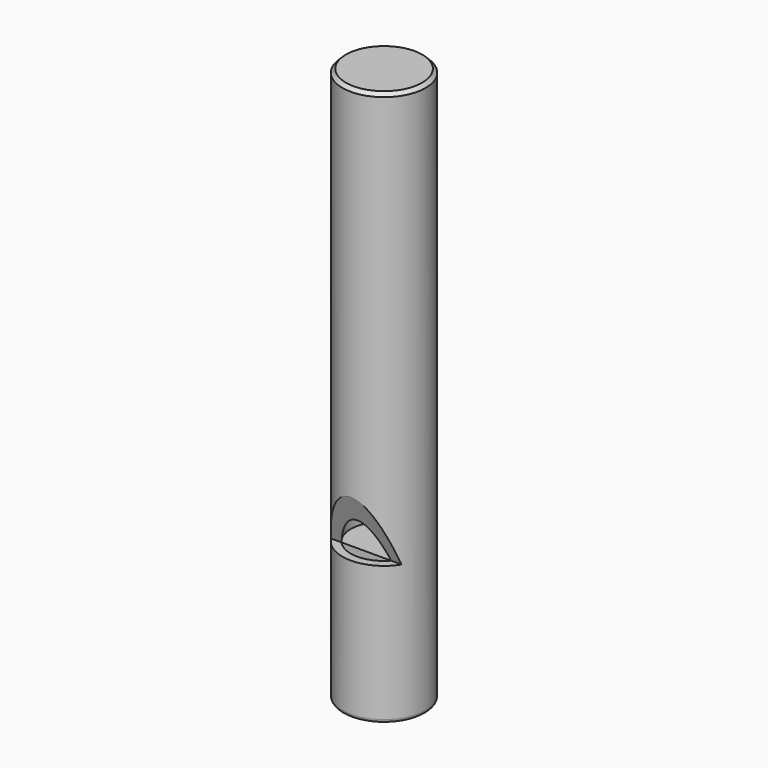
from build123d import *

# Parameters (mm, degrees)
F0_R     = 6
F0_R_2   = 4.8
F1_DEPTH = 80
F3_DEPTH = 12.5
F5_DEPTH = 15
F6_R     = 4.8
F7_DEPTH = 2
F8_R     = 0.5
F9_SIZE  = 0.5


with BuildPart() as f1:
    # F0 (on Top) → F1 (new body)
    with BuildSketch(Plane.XY):
        Circle(F0_R)
        Circle(F0_R_2, mode=Mode.SUBTRACT)
    extrude(amount=F1_DEPTH)

    # F2 (on Right) → F3 (cut, symmetric)
    with BuildSketch(Plane.YZ):
        Polygon((-6.6873627901, 30), (-6.6873627901, 20), (-3.1873627901, 20), align=None)
    extrude(amount=F3_DEPTH, both=True, mode=Mode.SUBTRACT)

    # F4 (on face) → F5 (join)
    with BuildSketch(Plane.XY.offset(20)):
        with BuildLine():
            Line((-3.5889717809, -3.1873627901), (3.5889717809, -3.1873627901))
            ThreePointArc((3.5889717809, -3.1873627901), (0, 4.8), (-3.5889717809, -3.1873627901))
        make_face()
    extrude(amount=-F5_DEPTH)

    # F6 (on face) → F7 (join)
    with BuildSketch(Plane.XY.offset(80)):
        Circle(F6_R)
    extrude(amount=-F7_DEPTH)

    # F8
    f8_edges = [f1.edges().sort_by_distance(p)[0] for p in [
        (-6, 0, 0),
    ]]
    fillet(f8_edges, radius=F8_R)

    # F9
    f9_edges = [f1.edges().sort_by_distance(p)[0] for p in [
        (-6, 0, 80),
    ]]
    chamfer(f9_edges, length=F9_SIZE)


solid = f1.part
